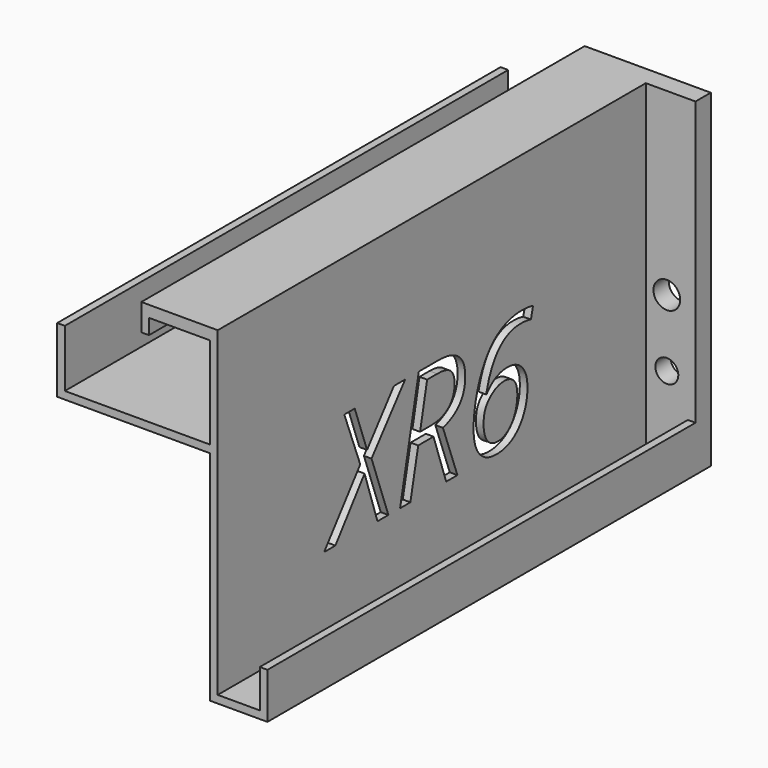
from build123d import *

# Parameters (mm, degrees)
F1_DEPTH      = 145
F2_W          = 11
F2_H          = 10
F3_DEPTH      = 140
F5_W          = 5
F5_H          = 69.6590341926
F6_DEPTH      = 13
F7_R          = 3.5
F7_R_2        = 3
F8_DEPTH      = 6
F9_W          = 13
F9_H          = 4.3409658074
F10_DEPTH     = 5
F11_TEXT_SIZE = 40.6085811038
F12_DEPTH     = 5


# Not quite as in the source:
# - Text() gives the source's letters only with a copy of the font that has no kerning and outlines rounded to 1/6400 em; it was checked with that copy


with BuildPart() as f1:
    # F0 (on Front) → F1 (new body)
    with BuildSketch(Plane.XZ):
        Polygon((0, 14), (0, -43), (15, -43), (15, -31), (2, -31), (2, 43), (-18, 43), (-18, 36), (-16, 36), (-16, 40), (0, 40), (0, 16), (-38, 16), (-38, 31), (-40, 31), (-40, 14), align=None)
    extrude(amount=F1_DEPTH)

    # F2 (on face) → F3 (cut)
    with BuildSketch(Plane.XZ.offset(145)):
        with Locations((7.5, -36)):
            Rectangle(F2_W, F2_H)
    extrude(amount=-F3_DEPTH, mode=Mode.SUBTRACT)

    # F5 (on face) → F6 (join)
    with BuildSketch(Plane.YZ.offset(2)):
        with Locations((-2.5, 8.1704829037)):
            Rectangle(F5_W, F5_H)
    extrude(amount=F6_DEPTH)

    # F7 (on face) → F8 (cut)
    with BuildSketch(Plane(origin=(0, 0, 0), x_dir=(-1, 0, 0), z_dir=(0, 1, 0))):
        with Locations((-7.5, -4)):
            Circle(F7_R)
        with Locations((-7.5, -21.5)):
            Circle(F7_R_2)
    extrude(amount=-F8_DEPTH, mode=Mode.SUBTRACT)

    # F9 (on face) → F10 (join)
    with BuildSketch(Plane(origin=(0, 0, 0), x_dir=(-1, 0, 0), z_dir=(0, 1, 0))):
        with Locations((-8.5, -28.8295170963)):
            Rectangle(F9_W, F9_H)
    extrude(amount=-F10_DEPTH)

    # F11 (on face) → F12 (cut)
    with BuildSketch(Plane.YZ.offset(2)):
        with Locations((-108.1493869424, -22.2511254251)):
            Text('XR6', F11_TEXT_SIZE, font='Open Sans', font_style=FontStyle.ITALIC, text_align=(TextAlign.LEFT, TextAlign.BOTTOM))
    extrude(amount=-F12_DEPTH, mode=Mode.SUBTRACT)


solid = f1.part
